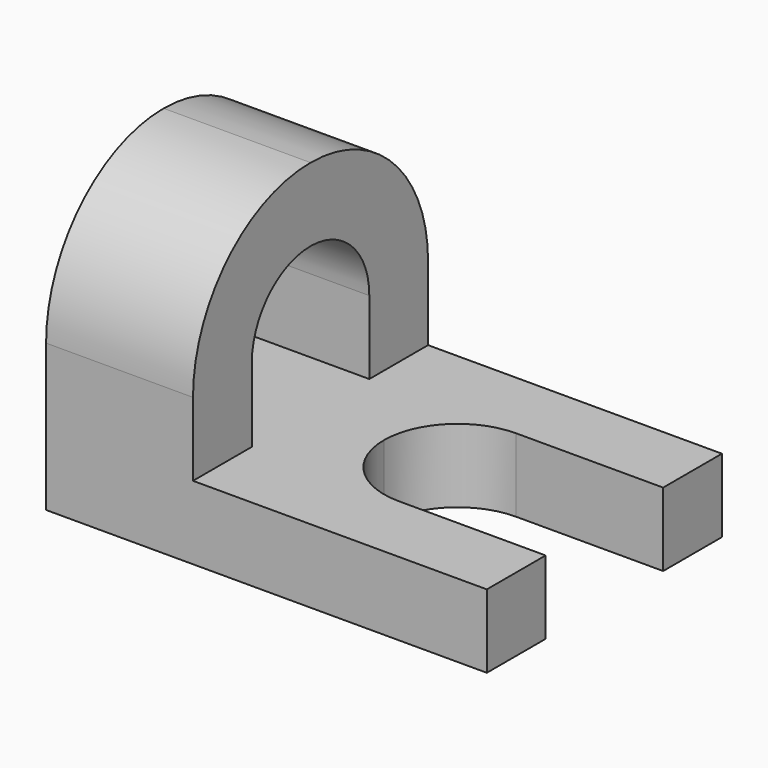
from build123d import *

# Parameters (mm, degrees)
F1_DEPTH = 50.8
F2_W     = 50.8
F2_H     = 50.8
F3_DEPTH = 204.4911384583
F4_W     = 76.2
F4_H     = 50.8
F5_DEPTH = 61.3817144185
F6_R     = 50.79999
F7_R     = 25.39999
F8_R     = 25.39999


# Not quite as in the source:
# - a fillet or chamfer is up to 0.001 mm smaller than in the source, because OpenCascade refuses the exact size


with BuildPart() as f1:
    # F0 (on Front) → F1 (new body, symmetric)
    with BuildSketch(Plane.XZ):
        Polygon((-25.4, -25.4), (-25.4, 50.8), (-76.2, 50.8), (-76.2, -50.8), (76.2, -50.8), (76.2, -25.4), align=None)
    extrude(amount=F1_DEPTH, both=True)

    # F2 (on face) → F3 (cut)
    with BuildSketch(Plane.YZ.offset(-25.4)):
        Rectangle(F2_W, F2_H)
    extrude(amount=-F3_DEPTH, mode=Mode.SUBTRACT)

    # F4 (on face) → F5 (cut)
    with BuildSketch(Plane.XY.offset(-25.4)):
        with Locations((38.1, 0)):
            Rectangle(F4_W, F4_H)
    extrude(amount=-F5_DEPTH, mode=Mode.SUBTRACT)

    # F6 (radius 50.8 in the source; OpenCascade refuses exactly that, so slightly less here)
    f6_edges = [f1.edges().sort_by_distance(p)[0] for p in [
        (-50.8, -50.8, 50.8),
        (-50.8, 50.8, 50.8),
    ]]
    fillet(f6_edges, radius=F6_R)

    # F7 (radius 25.4 in the source; OpenCascade refuses exactly that, so slightly less here)
    f7_edges = [f1.edges().sort_by_distance(p)[0] for p in [
        (-50.8, -25.4, 25.4),
        (-50.8, 25.4, 25.4),
    ]]
    fillet(f7_edges, radius=F7_R)

    # F8 (radius 25.4 in the source; OpenCascade refuses exactly that, so slightly less here)
    f8_edges = [f1.edges().sort_by_distance(p)[0] for p in [
        (0, -25.4, -38.1),
        (0, 25.4, -38.1),
    ]]
    fillet(f8_edges, radius=F8_R)


solid = f1.part
